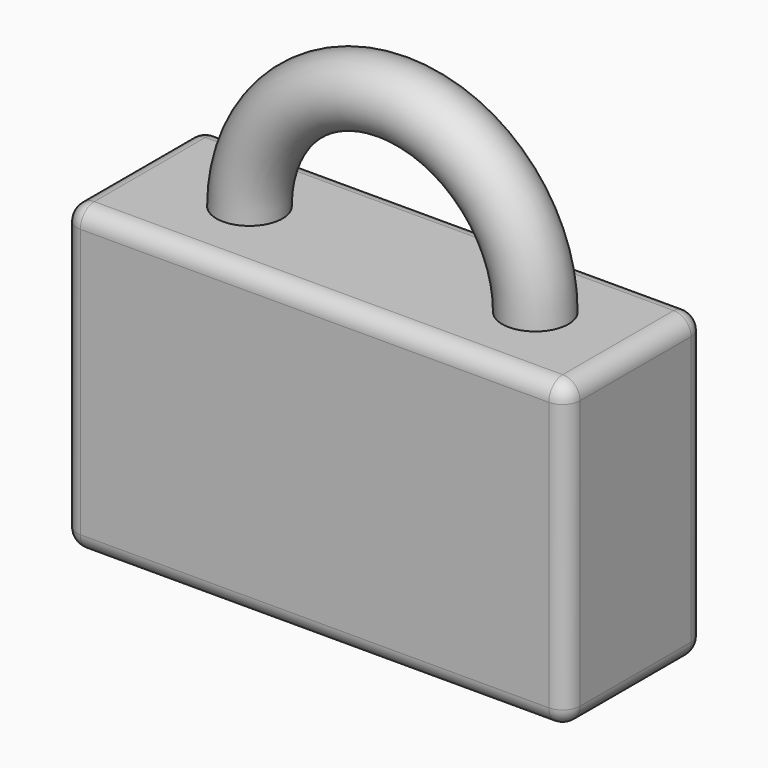
from build123d import *

# Parameters (mm, degrees)
F1_R         = 9.6860400986
F3_W         = 147.32
F3_H         = 88.9
F4_DEPTH     = 25.4
F5_R         = 5.08
F6_T1_DEPTH  = 40.64
F6_S5_W      = 5.08
F6_S5_H      = 5.08
F6_T6_DEPTH  = 5.08
F6_S11_W     = 5.08
F6_S11_H     = 5.08
F6_T12_DEPTH = 5.08
F7_T1_DEPTH  = 40.64
F7_S5_W      = 5.08
F7_S5_H      = 5.08
F7_T6_DEPTH  = 5.08
F7_S11_W     = 5.08
F7_S11_H     = 5.08
F7_T12_DEPTH = 5.08
F8_T1_DEPTH  = 40.64
F8_T3_DEPTH  = 137.16
F8_S7_W      = 5.08
F8_S7_H      = 5.08
F8_T8_DEPTH  = 5.08
F8_S13_W     = 5.08
F8_S13_H     = 5.08
F8_T14_DEPTH = 5.08
F8_T18_ANGLE = 90
F8_T20_ANGLE = 90


# Not quite as in the source:
# - a fillet or chamfer that OpenCascade refuses, or shapes differently, is made with other operations: its cross-section is extruded or revolved along the edge and cut away or added


with BuildPart() as f2:
    # F2: sweep along a path in F0
    with BuildLine(Plane.XZ) as f2_path:
        ThreePointArc((37.5847704709, 0), (-4.2709950358, 41.8557655066), (-46.1267605424, 0))
    # F1 (on Top) → F2 (sweep)
    with BuildSketch(Plane.XY):
        with Locations((37.5847704709, 0)):
            Circle(F1_R)
    sweep(path=f2_path.line)

    # F3 (on Front) → F4 (join, symmetric)
    with BuildSketch(Plane.XZ):
        with Locations((-6.7246720757, -44.45)):
            Rectangle(F3_W, F3_H)
    extrude(amount=F4_DEPTH, both=True)

    # F5
    f5_edges = [f2.edges().sort_by_distance(p)[0] for p in [
        (-80.384672, -25.4, -44.45),
        (66.935328, -25.4, -44.45),
        (66.935328, 25.4, -44.45),
        (-80.384672, 25.4, -44.45),
        (-6.724672, 25.4, 0),
        (-6.724672, -25.4, -88.9),
        (-6.724672, -25.4, 0),
    ]]
    fillet(f5_edges, radius=F5_R)

    # F6: fillet of radius 5.08 on 1 edges, made by hand

    # F6_s2 → F6_t1 (cut)
    with BuildSketch(Plane.XZ.offset(-20.32)):
        with BuildLine():
            ThreePointArc((61.8553279243, 0), (65.4474303727, -1.4878975516), (66.9353279243, -5.08))
            Line((66.9353279243, -5.08), (66.9353279243, 0))
            Line((66.9353279243, 0), (61.8553279243, 0))
        make_face()
    extrude(amount=F6_T1_DEPTH, mode=Mode.SUBTRACT)


with BuildPart() as f6_tool4:
    # F6_s5 → F6_t6 (new body)
    with BuildSketch(Plane.XY.offset(-5.08)):
        with Locations((64.3953279243, -22.86)):
            Rectangle(F6_S5_W, F6_S5_H)
    extrude(amount=F6_T6_DEPTH)

    # F6_s7 → F6_t8 (revolve, cut)
    with BuildSketch(Plane(origin=(61.8553279243, -20.32, -5.08), x_dir=(-0.7071067812, 0.7071067812, 0), z_dir=(0.7071067812, 0.7071067812, 0))):
        with BuildLine():
            ThreePointArc((0, -5.08), (5.08, 0), (0, 5.08))
            Line((0, 5.08), (0, -5.08))
        make_face()
    revolve(axis=Axis((61.8553279243, -20.32, -5.08), (0, 0, 1)), mode=Mode.SUBTRACT)


with BuildPart() as f2_1:
    add(f2.part)

    # F6_t3: cut F6_tool4
    add(f6_tool4.part, mode=Mode.SUBTRACT)


with BuildPart() as f6_tool10:
    # F6_s11 → F6_t12 (new body)
    with BuildSketch(Plane.XY.offset(-5.08)):
        with Locations((64.3953279243, 22.86)):
            Rectangle(F6_S11_W, F6_S11_H)
    extrude(amount=F6_T12_DEPTH)

    # F6_s13 → F6_t14 (revolve, cut)
    with BuildSketch(Plane(origin=(61.8553279243, 20.32, -5.08), x_dir=(-0.7071067812, -0.7071067812, 0), z_dir=(-0.7071067812, 0.7071067812, 0))):
        with BuildLine():
            ThreePointArc((0, -5.08), (5.08, 0), (0, 5.08))
            Line((0, 5.08), (0, -5.08))
        make_face()
    revolve(axis=Axis((61.8553279243, 20.32, -5.08), (0, 0, 1)), mode=Mode.SUBTRACT)


with BuildPart() as f2_2:
    add(f2_1.part)

    # F6_t9: cut F6_tool10
    add(f6_tool10.part, mode=Mode.SUBTRACT)

    # F7: fillet of radius 5.08 on 1 edges, made by hand

    # F7_s2 → F7_t1 (cut)
    with BuildSketch(Plane.XZ.offset(-20.32)):
        with BuildLine():
            ThreePointArc((-75.3046720757, 0), (-78.8967745241, -1.4878975516), (-80.3846720757, -5.08))
            Line((-80.3846720757, -5.08), (-80.3846720757, 0))
            Line((-80.3846720757, 0), (-75.3046720757, 0))
        make_face()
    extrude(amount=F7_T1_DEPTH, mode=Mode.SUBTRACT)


with BuildPart() as f7_tool4:
    # F7_s5 → F7_t6 (new body)
    with BuildSketch(Plane.XY.offset(-5.08)):
        with Locations((-77.8446720757, 22.86)):
            Rectangle(F7_S5_W, F7_S5_H)
    extrude(amount=F7_T6_DEPTH)

    # F7_s7 → F7_t8 (revolve, cut)
    with BuildSketch(Plane(origin=(-75.3046720757, 20.32, -5.08), x_dir=(0.7071067812, -0.7071067812, 0), z_dir=(-0.7071067812, -0.7071067812, 0))):
        with BuildLine():
            ThreePointArc((0, -5.08), (5.08, 0), (0, 5.08))
            Line((0, 5.08), (0, -5.08))
        make_face()
    revolve(axis=Axis((-75.3046720757, 20.32, -5.08), (0, 0, 1)), mode=Mode.SUBTRACT)


with BuildPart() as f2_3:
    add(f2_2.part)

    # F7_t3: cut F7_tool4
    add(f7_tool4.part, mode=Mode.SUBTRACT)


with BuildPart() as f7_tool10:
    # F7_s11 → F7_t12 (new body)
    with BuildSketch(Plane.XY.offset(-5.08)):
        with Locations((-77.8446720757, -22.86)):
            Rectangle(F7_S11_W, F7_S11_H)
    extrude(amount=F7_T12_DEPTH)

    # F7_s13 → F7_t14 (revolve, cut)
    with BuildSketch(Plane(origin=(-75.3046720757, -20.32, -5.08), x_dir=(0.7071067812, 0.7071067812, 0), z_dir=(0.7071067812, -0.7071067812, 0))):
        with BuildLine():
            ThreePointArc((0, -5.08), (5.08, 0), (0, 5.08))
            Line((0, 5.08), (0, -5.08))
        make_face()
    revolve(axis=Axis((-75.3046720757, -20.32, -5.08), (0, 0, 1)), mode=Mode.SUBTRACT)


with BuildPart() as f2_4:
    add(f2_3.part)

    # F7_t9: cut F7_tool10
    add(f7_tool10.part, mode=Mode.SUBTRACT)

    # F8: fillet of radius 5.08 on 1 edges, made by hand

    # F8_s2 → F8_t1 (cut)
    with BuildSketch(Plane.XZ.offset(-20.32)):
        with BuildLine():
            ThreePointArc((-80.3846720757, -83.82), (-78.8967745241, -87.4121024484), (-75.3046720757, -88.9))
            Line((-75.3046720757, -88.9), (-80.3846720757, -88.9))
            Line((-80.3846720757, -88.9), (-80.3846720757, -83.82))
        make_face()
        with BuildLine():
            ThreePointArc((66.9353279243, -83.82), (65.4474303727, -87.4121024484), (61.8553279243, -88.9))
            Line((61.8553279243, -88.9), (66.9353279243, -88.9))
            Line((66.9353279243, -88.9), (66.9353279243, -83.82))
        make_face()
    extrude(amount=F8_T1_DEPTH, mode=Mode.SUBTRACT)

    # F8_s4 → F8_t3 (cut)
    with BuildSketch(Plane.YZ.offset(-75.3046720757)):
        with BuildLine():
            ThreePointArc((25.4, -83.82), (23.9121024484, -87.4121024484), (20.32, -88.9))
            Line((20.32, -88.9), (25.4, -88.9))
            Line((25.4, -88.9), (25.4, -83.82))
        make_face()
    extrude(amount=F8_T3_DEPTH, mode=Mode.SUBTRACT)


with BuildPart() as f8_tool6:
    # F8_s7 → F8_t8 (new body)
    with BuildSketch(Plane.YZ.offset(-75.3046720757)):
        with Locations((-22.86, -86.36)):
            Rectangle(F8_S7_W, F8_S7_H)
    extrude(amount=-F8_T8_DEPTH)

    # F8_s9 → F8_t10 (revolve, cut)
    with BuildSketch(Plane(origin=(-75.3046720757, -20.32, -83.82), x_dir=(0, 0.7071067812, 0.7071067812), z_dir=(0, -0.7071067812, 0.7071067812))):
        with BuildLine():
            ThreePointArc((0, -5.08), (5.08, 0), (0, 5.08))
            Line((0, 5.08), (0, -5.08))
        make_face()
    revolve(axis=Axis((-75.3046720757, -20.32, -83.82), (-1, 0, 0)), mode=Mode.SUBTRACT)


with BuildPart() as f2_5:
    add(f2_4.part)

    # F8_t5: cut F8_tool6
    add(f8_tool6.part, mode=Mode.SUBTRACT)


with BuildPart() as f8_tool12:
    # F8_s13 → F8_t14 (new body)
    with BuildSketch(Plane.YZ.offset(61.8553279243)):
        with Locations((-22.86, -86.36)):
            Rectangle(F8_S13_W, F8_S13_H)
    extrude(amount=F8_T14_DEPTH)

    # F8_s15 → F8_t16 (revolve, cut)
    with BuildSketch(Plane(origin=(61.8553279243, -20.32, -83.82), x_dir=(0, 0.7071067812, 0.7071067812), z_dir=(0, 0.7071067812, -0.7071067812))):
        with BuildLine():
            ThreePointArc((0, -5.08), (5.08, 0), (0, 5.08))
            Line((0, 5.08), (0, -5.08))
        make_face()
    revolve(axis=Axis((61.8553279243, -20.32, -83.82), (1, 0, 0)), mode=Mode.SUBTRACT)


with BuildPart() as f2_6:
    add(f2_5.part)

    # F8_t11: cut F8_tool12
    add(f8_tool12.part, mode=Mode.SUBTRACT)

    # F8_s17 → F8_t18 (revolve, cut)
    with BuildSketch(Plane.YZ.offset(-75.3046720757)):
        with BuildLine():
            ThreePointArc((20.32, -88.9), (23.9121024484, -87.4121024484), (25.4, -83.82))
            Line((25.4, -83.82), (25.4, -88.9))
            Line((25.4, -88.9), (20.32, -88.9))
        make_face()
    revolve(axis=Axis((-75.3046720757, 20.32, -88.9), (0, 0, 1)), revolution_arc=F8_T18_ANGLE, mode=Mode.SUBTRACT)

    # F8_s19 → F8_t20 (revolve, cut)
    with BuildSketch(Plane.YZ.offset(61.8553279243)):
        with BuildLine():
            ThreePointArc((20.32, -88.9), (23.9121024484, -87.4121024484), (25.4, -83.82))
            Line((25.4, -83.82), (25.4, -88.9))
            Line((25.4, -88.9), (20.32, -88.9))
        make_face()
    revolve(axis=Axis((61.8553279243, 20.32, -88.9), (0, 0, -1)), revolution_arc=F8_T20_ANGLE, mode=Mode.SUBTRACT)


solid = f2_6.part
